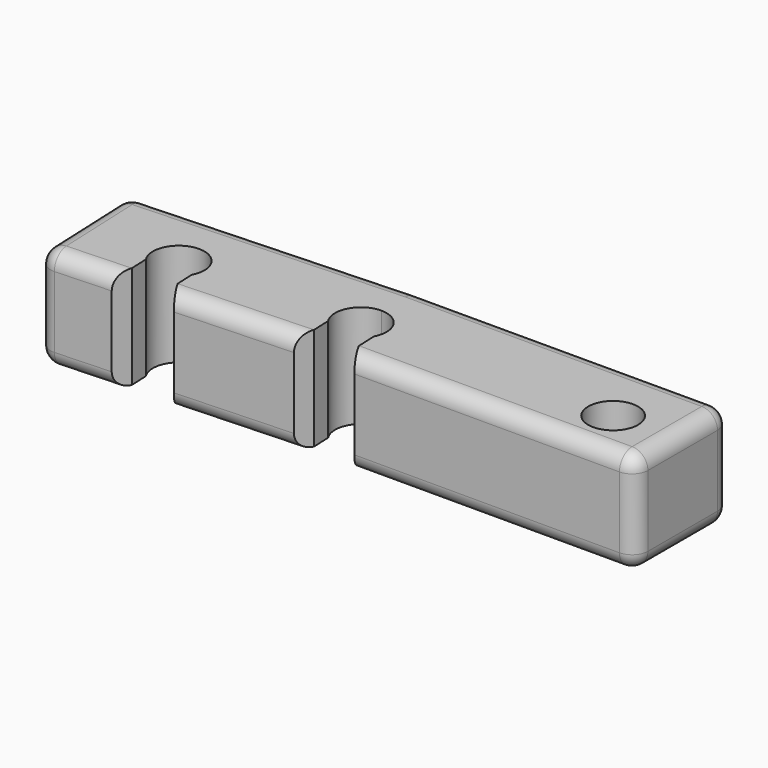
from build123d import *

# Parameters (mm, degrees)
F0_R        = 3.15
F1_DEPTH    = 6.5
F2_T1_DEPTH = 23.3593154951
F2_T3_DEPTH = 23.1607876028
F4_R        = 2


# Not quite as in the source:
# - a fillet or chamfer that OpenCascade refuses, or shapes differently, is made with other operations: its cross-section is extruded or revolved along the edge and cut away or added
# - two fillets or chamfers of one size are made in one step


with BuildPart() as f1:
    # F0 (on Top) → F1 (new body, symmetric)
    with BuildSketch(Plane.XY):
        with BuildLine():
            ThreePointArc((-2.7271020198, -1.7678842082), (-2.8555317961, 1.5519143538), (0, 3.25))
            Line((0, 3.25), (0, 9))
            Line((0, 9), (-35.4682957019, 7.5))
            Line((-35.4682957019, 7.5), (-34.834492885, -7.4866038177))
            Line((-34.834492885, -7.4866038177), (-24.8215810327, -7.0592907796))
            Line((-24.8215810327, -7.0592907796), (-25.0071863621, -2.7101377293))
            ThreePointArc((-25.0071863621, -2.7101377293), (-23.2018810758, 2.1742815392), (-19.0300843423, -0.9422535211))
            ThreePointArc((-19.0300843423, -0.9422535211), (-19.1270804103, -1.7303310583), (-19.4122789298, -2.4713683356))
            Line((-19.4122789298, -2.4713683356), (-19.2266736003, -6.8205213858))
            Line((-19.2266736003, -6.8205213858), (-2.5418620091, -6.1084770138))
            Line((-2.5418620091, -6.1084770138), (-2.7271020198, -1.7678842082))
        make_face()
        with BuildLine():
            ThreePointArc((3.25, 0), (3.153003932, -0.7880775372), (2.8678054126, -1.5291148144))
            Line((2.8678054126, -1.5291148144), (3.0586058071, -6))
            Line((3.0586058071, -6), (39.5, -6))
            Line((39.5, -6), (39.5, 9))
            Line((39.5, 9), (0, 9))
            Line((0, 9), (0, 3.25))
            ThreePointArc((0, 3.25), (2.2980970389, 2.2980970389), (3.25, 0))
        make_face()
        with Locations((31.9, 0)):
            Circle(F0_R, mode=Mode.SUBTRACT)
    extrude(amount=F1_DEPTH, both=True)

    # F2: chamfer of 2 x 1 on 4 edges, made by hand

    # F2_s2 → F2_t1 (cut)
    with BuildSketch(Plane.XY.offset(-11.6796577476)):
        Polygon((-24.9068558162, -5.0611095538), (-25.8206716456, -7.1019281713), (-24.8215810327, -7.0592907796), align=None)
        Polygon((-2.6271367926, -4.110295788), (-3.540952622, -6.1511144056), (-2.5418620091, -6.1084770138), align=None)
        Polygon((-18.2275829874, -6.7778839941), (-19.3119483838, -4.82234016), (-19.2266736003, -6.8205213858), align=None)
    extrude(amount=F2_T1_DEPTH, mode=Mode.SUBTRACT)

    # F2_s4 → F2_t3 (cut)
    with BuildSketch(Plane.XY.offset(-11.5803938014)):
        Polygon((3.97416362, -6), (2.9750730071, -4.0426373917), (3.0586058071, -6), align=None)
    extrude(amount=F2_T3_DEPTH, mode=Mode.SUBTRACT)

    # F4
    f4_edges = [f1.edges().sort_by_distance(p)[0] for p in [
        (-17.734148, 8.25, 6.5),
        (19.75, 9, 6.5),
        (-17.734148, 8.25, -6.5),
        (19.75, 9, -6.5),
        (-35.468296, 7.5, 0),
        (39.5, 9, 0),
        (39.5, 1.5, 6.5),
        (39.5, 1.5, -6.5),
        (-35.151394, 0.006698, -6.5),
        (-35.151394, 0.006698, 6.5),
        (-34.834493, -7.486604, 0),
        (-30.327582, -7.294266, -6.5),
        (-30.327582, -7.294266, 6.5),
        (-10.884268, -6.464499, 6.5),
        (-10.884268, -6.464499, -6.5),
        (21.737082, -6, 6.5),
        (39.5, -6, 0),
        (21.737082, -6, -6.5),
    ]]
    fillet(f4_edges, radius=F4_R)


solid = f1.part
